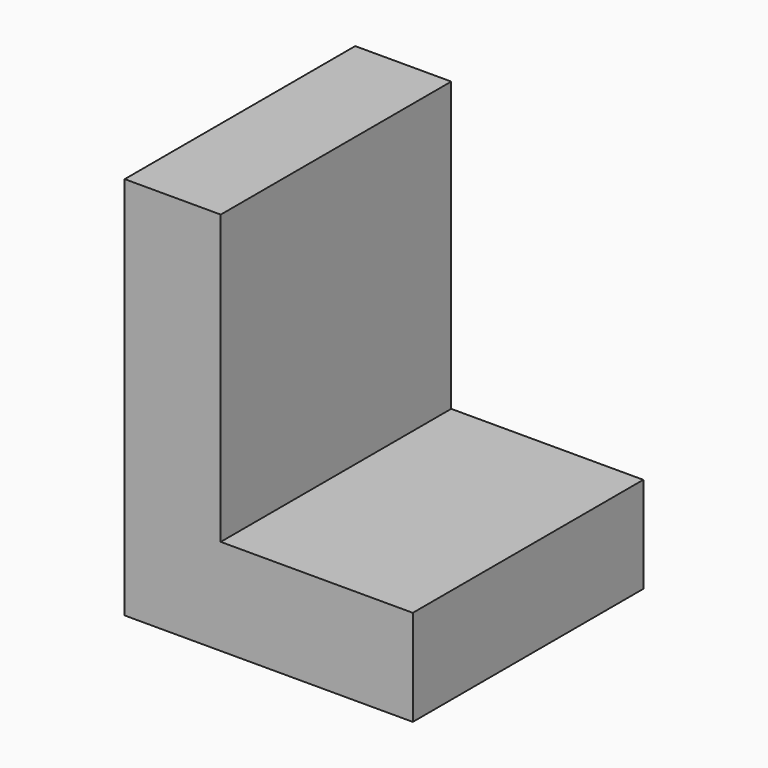
from build123d import *

# Parameters (mm, degrees)
F1_DEPTH = 152.4


# Not quite as in the source:
# - a feature names something its author has since deleted; it is built from what else it names


with BuildPart() as f1:
    # F0 (on Front) → F1 (new body)
    with BuildSketch(Plane.XZ):
        Polygon((50.8, 0), (0, 0), (0, -203.2), (152.4, -203.2), (152.4, -152.4), (50.8, -152.4), align=None)
    extrude(amount=F1_DEPTH)


solid = f1.part
